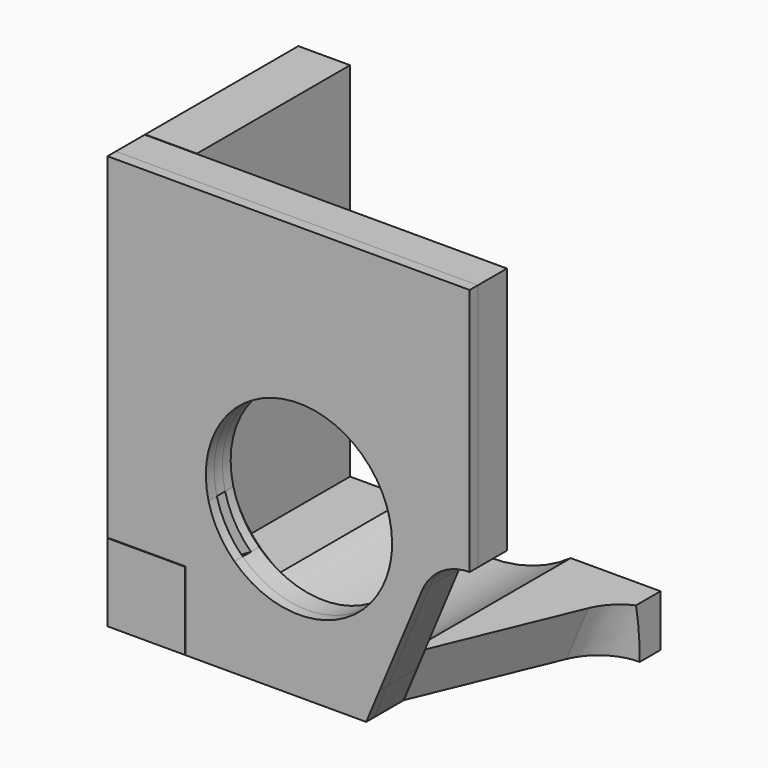
from build123d import *
from build123d import SkipClean  # not in build123d's __all__

# Parameters (mm, degrees)
F3_DEPTH       = 2
F4_DEPTH       = 5
F5_START       = 2
F5_DEPTH       = 2
F6_SIZE        = 3
F7_W           = 15
F7_H           = 15
F8_DEPTH       = 4
F9_START       = 2
F9_DEPTH       = 2
F2_W           = 10
F2_H           = 10
F10_DEPTH      = 5.1
F10_DEPTH_BACK = 2
F11_W          = 10
F11_H          = 10
F12_DEPTH      = 37


with BuildPart() as f3:
    # F2 (on Front) → F3 (new body)
    with BuildSketch(Plane.XZ):
        with BuildLine():
            Line((0, 0), (0, 48))
            Line((0, 48), (-70, 48))
            Line((-70, 48), (-70, -21.9))
            Line((-70, -21.9), (-59.9, -21.9))
            Line((-59.9, -21.9), (-59.9, -32))
            Line((-59.9, -32), (-26.6666666667, -32))
            Line((-26.6666666667, -32), (-20, -32))
            Line((-20, -32), (-17.4358974359, -25.8461538462))
            Line((-17.4358974359, -25.8461538462), (-9.2307692308, -6.1538461538))
            ThreePointArc((-9.2307692308, -6.1538461538), (-5.5470019623, -1.6794970566), (0, 0))
        make_face()
        with BuildLine():
            ThreePointArc((-28, 17.2916164658), (-18.6125054301, 10.8166538264), (-15, 0))
            ThreePointArc((-15, 0), (-15.1317372924, -2.1737497126), (-15.5250208681, -4.315681214))
            Line((-15.5250208681, -4.315681214), (-13.1794919243, -5.6698729811))
            Line((-13.1794919243, -5.6698729811), (-15.6794919243, -10))
            Line((-15.6794919243, -10), (-18.1794919243, -14.3301270189))
            Line((-18.1794919243, -14.3301270189), (-20.5250208681, -12.9759352518))
            ThreePointArc((-20.5250208681, -12.9759352518), (-33, -18), (-45.4749791319, -12.9759352518))
            Line((-45.4749791319, -12.9759352518), (-47.8205080757, -14.3301270189))
            Line((-47.8205080757, -14.3301270189), (-50.3205080757, -10))
            Line((-50.3205080757, -10), (-52.8205080757, -5.6698729811))
            Line((-52.8205080757, -5.6698729811), (-50.4749791319, -4.315681214))
            ThreePointArc((-50.4749791319, -4.315681214), (-48.5884572681, 9), (-38, 17.2916164658))
            Line((-38, 17.2916164658), (-38, 20))
            Line((-38, 20), (-33, 20))
            Line((-33, 20), (-28, 20))
            Line((-28, 20), (-28, 17.2916164658))
        make_face(mode=Mode.SUBTRACT)
    extrude(amount=F3_DEPTH)

    # F2 (on Front) → F4 (join)
    with BuildSketch(Plane.XZ):
        with BuildLine():
            Line((0, 0), (0, 48))
            Line((0, 48), (-70, 48))
            Line((-70, 48), (-70, -21.9))
            Line((-70, -21.9), (-59.9, -21.9))
            Line((-59.9, -21.9), (-59.9, -32))
            Line((-59.9, -32), (-26.6666666667, -32))
            Line((-26.6666666667, -32), (-20, -32))
            Line((-20, -32), (-17.4358974359, -25.8461538462))
            Line((-17.4358974359, -25.8461538462), (-9.2307692308, -6.1538461538))
            ThreePointArc((-9.2307692308, -6.1538461538), (-5.5470019623, -1.6794970566), (0, 0))
        make_face()
        with BuildLine():
            ThreePointArc((-28, 17.2916164658), (-18.6125054301, 10.8166538264), (-15, 0))
            ThreePointArc((-15, 0), (-15.1317372924, -2.1737497126), (-15.5250208681, -4.315681214))
            Line((-15.5250208681, -4.315681214), (-13.1794919243, -5.6698729811))
            Line((-13.1794919243, -5.6698729811), (-15.6794919243, -10))
            Line((-15.6794919243, -10), (-18.1794919243, -14.3301270189))
            Line((-18.1794919243, -14.3301270189), (-20.5250208681, -12.9759352518))
            ThreePointArc((-20.5250208681, -12.9759352518), (-33, -18), (-45.4749791319, -12.9759352518))
            Line((-45.4749791319, -12.9759352518), (-47.8205080757, -14.3301270189))
            Line((-47.8205080757, -14.3301270189), (-50.3205080757, -10))
            Line((-50.3205080757, -10), (-52.8205080757, -5.6698729811))
            Line((-52.8205080757, -5.6698729811), (-50.4749791319, -4.315681214))
            ThreePointArc((-50.4749791319, -4.315681214), (-48.5884572681, 9), (-38, 17.2916164658))
            Line((-38, 17.2916164658), (-38, 20))
            Line((-38, 20), (-33, 20))
            Line((-33, 20), (-28, 20))
            Line((-28, 20), (-28, 17.2916164658))
        make_face(mode=Mode.SUBTRACT)
        with BuildLine():
            ThreePointArc((-45.4749791319, -12.9759352518), (-48.5884572681, -9), (-50.4749791319, -4.315681214))
            Line((-50.4749791319, -4.315681214), (-52.8205080757, -5.6698729811))
            Line((-52.8205080757, -5.6698729811), (-50.3205080757, -10))
            Line((-50.3205080757, -10), (-47.8205080757, -14.3301270189))
            Line((-47.8205080757, -14.3301270189), (-45.4749791319, -12.9759352518))
        make_face()
        with BuildLine():
            Line((-13.1794919243, -5.6698729811), (-15.5250208681, -4.315681214))
            ThreePointArc((-15.5250208681, -4.315681214), (-17.4115427319, -9), (-20.5250208681, -12.9759352518))
            Line((-20.5250208681, -12.9759352518), (-18.1794919243, -14.3301270189))
            Line((-18.1794919243, -14.3301270189), (-15.6794919243, -10))
            Line((-15.6794919243, -10), (-13.1794919243, -5.6698729811))
        make_face()
        with BuildLine():
            ThreePointArc((-38, 17.2916164658), (-33, 18), (-28, 17.2916164658))
            Line((-28, 17.2916164658), (-28, 20))
            Line((-28, 20), (-33, 20))
            Line((-33, 20), (-38, 20))
            Line((-38, 20), (-38, 17.2916164658))
        make_face()
    with SkipClean():  # cleaning this boolean's faces spoils the solid; the shape is the same uncleaned
        extrude(amount=-F4_DEPTH)

    # F6
    f6_edges = [f3.edges().sort_by_distance(p)[0] for p in [
        (-28, 5, -17.291616),
    ]]
    chamfer(f6_edges, length=F6_SIZE)


with BuildPart() as f5:
    # F2 (on Front) → F5 (new body)
    with BuildSketch(Plane.XZ.offset(F5_START)):
        with BuildLine():
            Line((0, 0), (0, 48))
            Line((0, 48), (-70, 48))
            Line((-70, 48), (-70, -21.9))
            Line((-70, -21.9), (-59.9, -21.9))
            Line((-59.9, -21.9), (-59.9, -32))
            Line((-59.9, -32), (-26.6666666667, -32))
            Line((-26.6666666667, -32), (-20, -32))
            Line((-20, -32), (-17.4358974359, -25.8461538462))
            Line((-17.4358974359, -25.8461538462), (-9.2307692308, -6.1538461538))
            ThreePointArc((-9.2307692308, -6.1538461538), (-5.5470019623, -1.6794970566), (0, 0))
        make_face()
        with BuildLine():
            ThreePointArc((-28, 17.2916164658), (-18.6125054301, 10.8166538264), (-15, 0))
            ThreePointArc((-15, 0), (-15.1317372924, -2.1737497126), (-15.5250208681, -4.315681214))
            Line((-15.5250208681, -4.315681214), (-13.1794919243, -5.6698729811))
            Line((-13.1794919243, -5.6698729811), (-15.6794919243, -10))
            Line((-15.6794919243, -10), (-18.1794919243, -14.3301270189))
            Line((-18.1794919243, -14.3301270189), (-20.5250208681, -12.9759352518))
            ThreePointArc((-20.5250208681, -12.9759352518), (-33, -18), (-45.4749791319, -12.9759352518))
            Line((-45.4749791319, -12.9759352518), (-47.8205080757, -14.3301270189))
            Line((-47.8205080757, -14.3301270189), (-50.3205080757, -10))
            Line((-50.3205080757, -10), (-52.8205080757, -5.6698729811))
            Line((-52.8205080757, -5.6698729811), (-50.4749791319, -4.315681214))
            ThreePointArc((-50.4749791319, -4.315681214), (-48.5884572681, 9), (-38, 17.2916164658))
            Line((-38, 17.2916164658), (-38, 20))
            Line((-38, 20), (-33, 20))
            Line((-33, 20), (-28, 20))
            Line((-28, 20), (-28, 17.2916164658))
        make_face(mode=Mode.SUBTRACT)
        with BuildLine():
            ThreePointArc((-45.4749791319, -12.9759352518), (-48.5884572681, -9), (-50.4749791319, -4.315681214))
            Line((-50.4749791319, -4.315681214), (-52.8205080757, -5.6698729811))
            Line((-52.8205080757, -5.6698729811), (-50.3205080757, -10))
            Line((-50.3205080757, -10), (-47.8205080757, -14.3301270189))
            Line((-47.8205080757, -14.3301270189), (-45.4749791319, -12.9759352518))
        make_face()
        with BuildLine():
            Line((-13.1794919243, -5.6698729811), (-15.5250208681, -4.315681214))
            ThreePointArc((-15.5250208681, -4.315681214), (-17.4115427319, -9), (-20.5250208681, -12.9759352518))
            Line((-20.5250208681, -12.9759352518), (-18.1794919243, -14.3301270189))
            Line((-18.1794919243, -14.3301270189), (-15.6794919243, -10))
            Line((-15.6794919243, -10), (-13.1794919243, -5.6698729811))
        make_face()
        with BuildLine():
            ThreePointArc((-38, 17.2916164658), (-33, 18), (-28, 17.2916164658))
            Line((-28, 17.2916164658), (-28, 20))
            Line((-28, 20), (-33, 20))
            Line((-33, 20), (-38, 20))
            Line((-38, 20), (-38, 17.2916164658))
        make_face()
    extrude(amount=F5_DEPTH)

    # F7 (on Front) → F8 (cut)
    with BuildSketch(Plane.XZ):
        with Locations((-62.5, -24.5)):
            Rectangle(F7_W, F7_H)
        Polygon((-55, -17), (-55, -32), (-54.9, -32), (-54.9, -16.9), (-70, -16.9), (-70, -17), align=None)
    extrude(amount=F8_DEPTH, mode=Mode.SUBTRACT)


with BuildPart() as f9:
    # F7 (on Front) → F9 (new body)
    with BuildSketch(Plane.XZ.offset(F9_START)):
        with Locations((-62.5, -24.5)):
            Rectangle(F7_W, F7_H)
    extrude(amount=F9_DEPTH)

    # F2 (on Front) → F10 (join, two sides)
    with BuildSketch(Plane.XZ) as f10_sk:
        with Locations((-65, -27)):
            Rectangle(F2_W, F2_H)
    extrude(amount=-F10_DEPTH)
    extrude(f10_sk.sketch, amount=F10_DEPTH_BACK)

    # F11 (on face) → F12 (join)
    with BuildSketch(Plane(origin=(0, 5.1, 0), x_dir=(-1, 0, 0), z_dir=(0, 1, 0))):
        with BuildLine():
            Line((0, -32), (60, -32))
            Line((60, -32), (60, -22))
            Line((60, -22), (48.6524758425, -22))
            ThreePointArc((48.6524758425, -22), (33, -27), (17.3475241575, -22))
            Line((17.3475241575, -22), (0, -22))
            Line((0, -22), (0, -32))
        make_face()
        Polygon((60, -22), (70, -22), (70, 48), (60, 48), (60, 0), align=None)
        with Locations((65, -27)):
            Rectangle(F11_W, F11_H)
    extrude(amount=F12_DEPTH)

    # F14: sweep along a path in F14_path
    with BuildLine(Plane(origin=(-20, 5, -32), x_dir=(-0.3846153846, 0, -0.9230769231), z_dir=(-0.9230769231, 0, 0.3846153846))) as f14_path:
        Line((0, 0), (-28, 0))
    # F13 (on face) → F14 (sweep, cut)
    with BuildSketch(Plane(origin=(0, 0, -32), x_dir=(1, 0, 0), z_dir=(0, 0, -1))):
        with BuildLine():
            Line((0, -5.1), (-20, -5.1))
            Line((-20, -5.1), (-9.2307692308, -30.9461538462))
            ThreePointArc((-9.2307692308, -30.9461538462), (-5.5470019623, -35.4205029434), (0, -37.1))
            Line((0, -37.1), (0, -5.1))
        make_face()
    sweep(path=f14_path.line, mode=Mode.SUBTRACT)


solid = Compound([f3.part, f5.part, f9.part])
